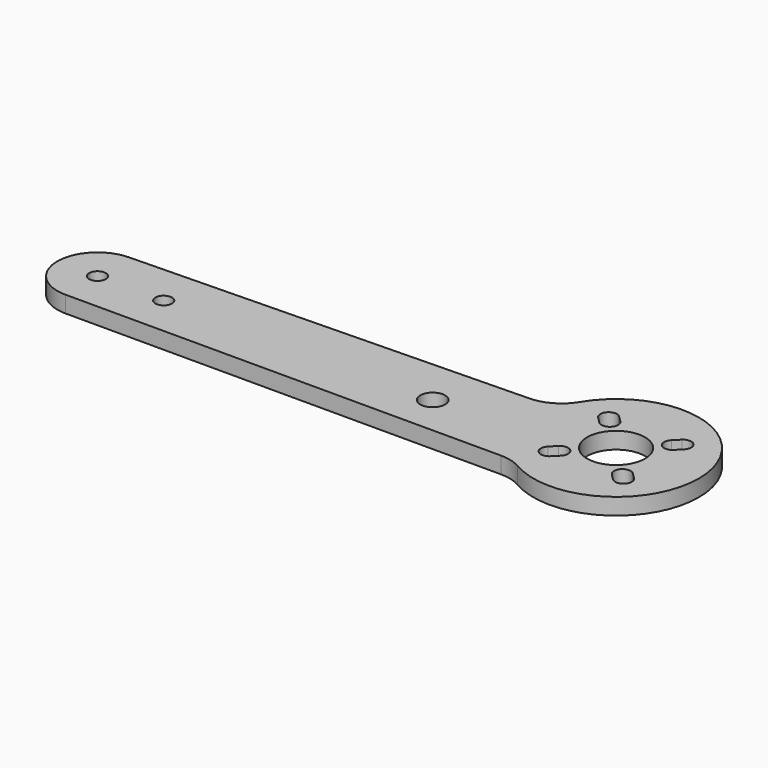
from build123d import *

# Parameters (mm, degrees)
F0_R     = 1
F0_R_2   = 1.5
F0_R_3   = 3.5
F1_DEPTH = 2


# Not quite as in the source:
# - ends of sketch curves that miss each other by under 0.0002 mm in the source are joined


with BuildPart() as f1:
    # F0 (on Top) → F1 (new body)
    with BuildSketch(Plane.XY):
        with BuildLine():
            ThreePointArc((-55.949488929, -12.7158224136), (-54.6584944803, -12.8853634982), (-53.4550506712, -13.3824890802))
            ThreePointArc((-53.4550506712, -13.3824890802), (-38.7798788654, -2.230730151), (-57.0112213811, 0.4786138322))
            ThreePointArc((-57.0112213811, 0.4786138322), (-58.7831707533, -1.2539634751), (-61.1694240668, -1.9228609466))
            Line((-61.1694240668, -1.9228609466), (-108.7206725135, -3.0103658035))
            ThreePointArc((-108.7206725135, -3.0103658035), (-108.7222436347, -3.0104019898), (-108.7238147676, -3.0104376674))
            ThreePointArc((-108.7238147676, -3.0104376674), (-113.4658569564, -7.9179829708), (-108.6128474049, -12.7158224136))
            Line((-108.6128474049, -12.7158224136), (-55.949488929, -12.7158224136))
        make_face()
        with Locations((-108.6128474049, -7.862495663)):
            Circle(F0_R, mode=Mode.SUBTRACT)
        with Locations((-100.6128474049, -7.862495663)):
            Circle(F0_R, mode=Mode.SUBTRACT)
        with Locations((-68.1128474049, -7.862495663)):
            Circle(F0_R_2, mode=Mode.SUBTRACT)
        with BuildLine():
            ThreePointArc((-52.2491954348, -9.9130572553), (-53.6634089972, -9.9130572553), (-53.6634089972, -8.4988436929))
            Line((-53.6634089972, -8.4988436929), (-52.956302216, -7.7917369117))
            ThreePointArc((-52.956302216, -7.7917369117), (-51.5420886536, -7.7917369117), (-51.5420886536, -9.2059504741))
            Line((-51.5420886536, -9.2059504741), (-52.2491954348, -9.9130572553))
        make_face(mode=Mode.SUBTRACT)
        with BuildLine():
            ThreePointArc((-43.2689393138, -8.4988436929), (-43.2689393138, -9.9130572553), (-44.6831528761, -9.9130572553))
            Line((-44.6831528761, -9.9130572553), (-45.3902596573, -9.2059504741))
            ThreePointArc((-45.3902596573, -9.2059504741), (-45.3902596573, -7.7917369117), (-43.9760460949, -7.7917369117))
            Line((-43.9760460949, -7.7917369117), (-43.2689393138, -8.4988436929))
        make_face(mode=Mode.SUBTRACT)
        with Locations((-48.4661741555, -4.7158224136)):
            Circle(F0_R_3, mode=Mode.SUBTRACT)
        with BuildLine():
            ThreePointArc((-53.6634089972, -0.9328011342), (-53.6634089972, 0.4814124282), (-52.2491954348, 0.4814124282))
            Line((-52.2491954348, 0.4814124282), (-51.5420886536, -0.225694353))
            ThreePointArc((-51.5420886536, -0.225694353), (-51.5420886536, -1.6399079154), (-52.956302216, -1.6399079154))
            Line((-52.956302216, -1.6399079154), (-53.6634089972, -0.9328011342))
        make_face(mode=Mode.SUBTRACT)
        with BuildLine():
            ThreePointArc((-43.9760460949, -1.6399079154), (-45.3902596573, -1.6399079154), (-45.3902596573, -0.225694353))
            Line((-45.3902596573, -0.225694353), (-44.6831528761, 0.4814124282))
            ThreePointArc((-44.6831528761, 0.4814124282), (-43.2689393138, 0.4814124282), (-43.2689393138, -0.9328011342))
            Line((-43.2689393138, -0.9328011342), (-43.9760460949, -1.6399079154))
        make_face(mode=Mode.SUBTRACT)
    extrude(amount=F1_DEPTH)


solid = f1.part
